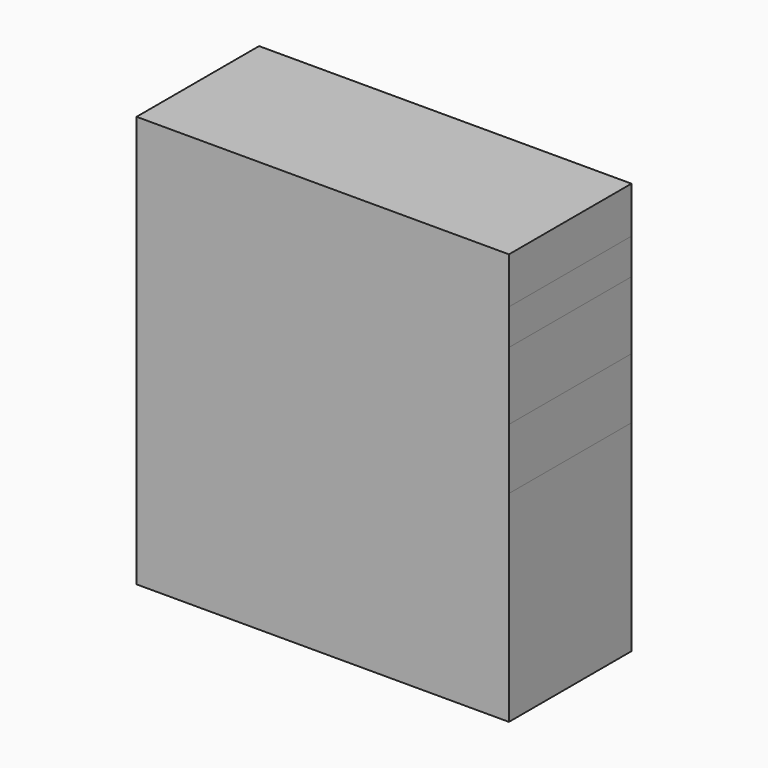
from build123d import *

# Parameters (mm, degrees)
F0_W     = 60.8069598675
F0_H     = 7.9524954781
F0_W_2   = 60.8069561422
F0_H_2   = 32.8389271162
F1_DEPTH = 25


# Not quite as in the source:
# - ends of sketch curves that miss each other by under 0.0002 mm in the source are joined


with BuildPart() as f1:
    # F0 (on Front) → F1 (new body)
    with BuildSketch(Plane.XZ):
        Polygon((60.8069561422, 67.2151967883), (0, 67.2151967883), (0, 62.0886087418), (0, 59.6657376736), (60.8069561422, 59.6657376736), (60.8069561422, 62.0886087418), align=None)
        Polygon((60.8069561422, 59.6657376736), (0, 59.6657376736), (0, 53.8291148841), (0, 50.7177971303), (60.8069598675, 50.7177971303), (60.8069598675, 53.8291148841), align=None)
        with Locations((30.4034799337, 46.7415493913)):
            Rectangle(F0_W, F0_H)
        Polygon((60.8069598675, 42.7653016523), (0, 42.7653016523), (0, 32.8389271162), (60.8069561422, 32.8389271162), align=None)
        with Locations((30.4034780711, 16.4194635581)):
            Rectangle(F0_W_2, F0_H_2)
    extrude(amount=F1_DEPTH)


solid = f1.part
